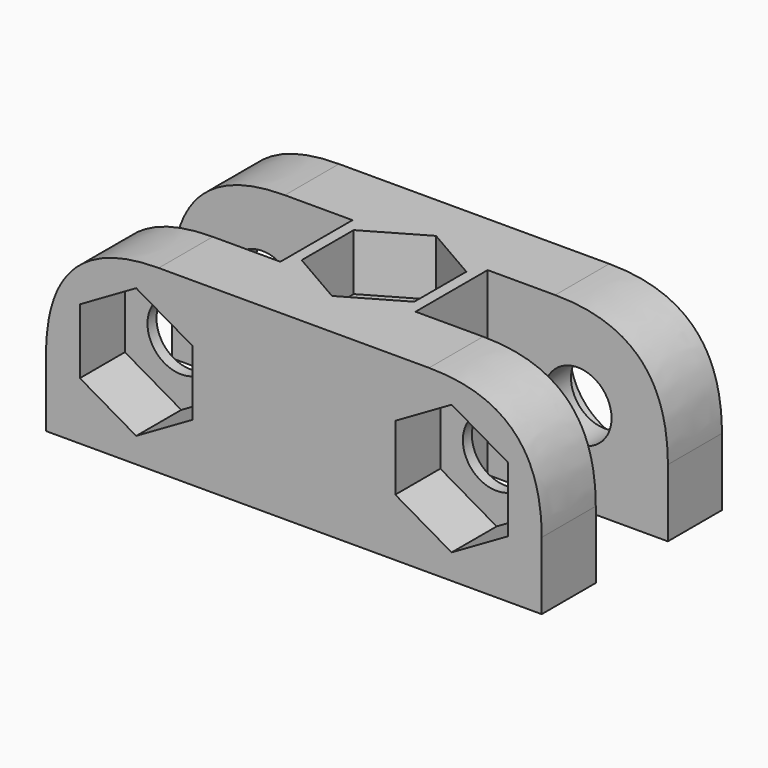
from build123d import *

# Parameters (mm, degrees)
F0_W        = 44
F0_H        = 20
F1_DEPTH    = 16
F2_R        = 3
F3_DEPTH    = 16
F5_DEPTH    = 5
F6_T1_DEPTH = 70
F7_R        = 3
F8_DEPTH    = 20
F10_DEPTH   = 5
F11_R       = 5.5
F12_DEPTH   = 3
F13_W       = 16
F13_H       = 8
F14_DEPTH   = 25


# Not quite as in the source:
# - a fillet or chamfer that OpenCascade refuses, or shapes differently, is made with other operations: its cross-section is extruded or revolved along the edge and cut away or added


with BuildPart() as f1:
    # F0 (on Top) → F1 (new body)
    with BuildSketch(Plane.XY):
        Rectangle(F0_W, F0_H)
    extrude(amount=F1_DEPTH)

    # F2 (on face) → F3 (cut, through all)
    with BuildSketch(Plane.XY.offset(16)):
        Circle(F2_R)
    extrude(amount=-F3_DEPTH, mode=Mode.SUBTRACT)

    # F4 (on face) → F5 (cut)
    with BuildSketch(Plane.XY.offset(16)):
        Polygon((5, -2.8867513459), (5, 2.8867513459), (0, 5.7735026919), (-5, 2.8867513459), (-5, -2.8867513459), (0, -5.7735026919), align=None)
    extrude(amount=-F5_DEPTH, mode=Mode.SUBTRACT)

    # F6: fillet of radius 10 on 2 edges, made by hand

    # F6_s2 → F6_t1 (cut)
    with BuildSketch(Plane.XZ.offset(-35)):
        with BuildLine():
            add(Edge.make_bspline(
                [(22, 6), (22, 16), (12, 16)],
                knots=[0, 0, 0, 1, 1, 1], degree=2, weights=[1, 1, 1]))
            Line((12, 16), (22, 16))
            Line((22, 16), (22, 6))
        make_face()
        with BuildLine():
            add(Edge.make_bspline(
                [(-22, 6), (-22, 16), (-12, 16)],
                knots=[0, 0, 0, 1, 1, 1], degree=2, weights=[1, 1, 1]))
            Line((-12, 16), (-22, 16))
            Line((-22, 16), (-22, 6))
        make_face()
    extrude(amount=F6_T1_DEPTH, mode=Mode.SUBTRACT)

    # F7 (on face) → F8 (cut, through all)
    with BuildSketch(Plane.XZ.offset(10)):
        with Locations((14, 8)):
            Circle(F7_R)
        with Locations((-14, 8)):
            Circle(F7_R)
    extrude(amount=-F8_DEPTH, mode=Mode.SUBTRACT)

    # F9 (on face) → F10 (cut)
    with BuildSketch(Plane.XZ.offset(10)):
        Polygon((9, 10.8867513459), (9, 5.1132486541), (14, 2.2264973081), (19, 5.1132486541), (19, 10.8867513459), (14, 13.7735026919), align=None)
        Polygon((-9, 5.1132486541), (-9, 10.8867513459), (-14, 13.7735026919), (-19, 10.8867513459), (-19, 5.1132486541), (-14, 2.2264973081), align=None)
    extrude(amount=-F10_DEPTH, mode=Mode.SUBTRACT)

    # F11 (on face) → F12 (cut)
    with BuildSketch(Plane(origin=(0, 10, 0), x_dir=(-1, 0, 0), z_dir=(0, 1, 0))):
        with Locations((-14, 8)):
            Circle(F11_R)
        with Locations((14, 8)):
            Circle(F11_R)
    extrude(amount=-F12_DEPTH, mode=Mode.SUBTRACT)

    # F13 (on face) → F14 (cut)
    with BuildSketch(Plane(origin=(0, 0, 0), x_dir=(1, 0, 0), z_dir=(0, 0, -1))):
        with Locations((-14, 0)):
            Rectangle(F13_W, F13_H)
        with Locations((14, 0)):
            Rectangle(F13_W, F13_H)
    extrude(amount=-F14_DEPTH, mode=Mode.SUBTRACT)


solid = f1.part
